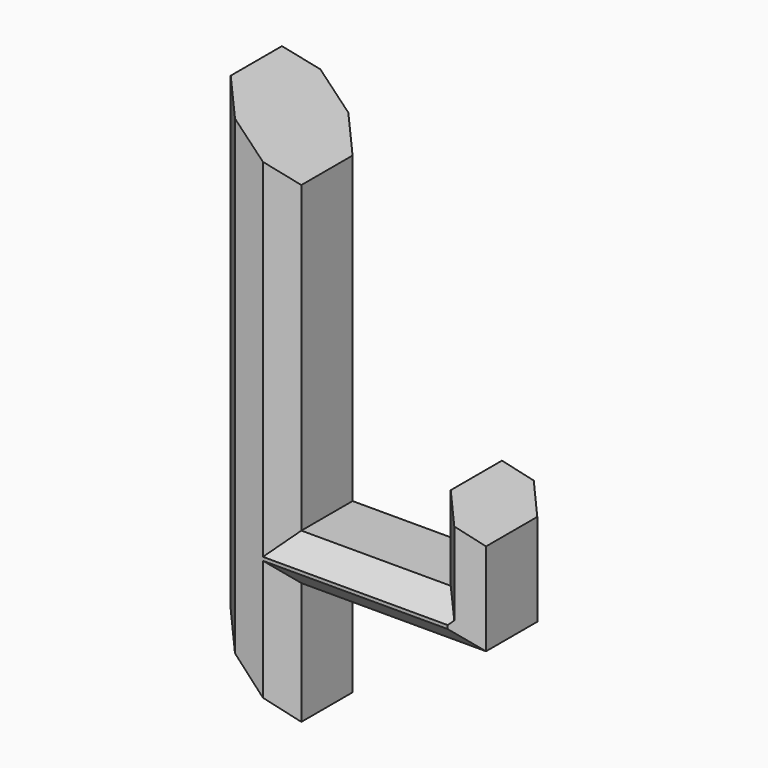
from build123d import *

# Parameters (mm, degrees)
F1_DEPTH   = 25
F2_SIZE    = 5
F3_SIZE    = 5
F4_C1_SIZE = 5
F4_C2_SIZE = 5
F4_C3_SIZE = 5
F4_C4_SIZE = 5
F5_SIZE    = 5
F6_R       = 3.8134977221
F6_R_2     = 4.2636207358
F6_R_3     = 3.889016134
F6_R_4     = 3.7558552916
F6_R_5     = 4.5761931688
F6_R_6     = 1.7054444875
F7_DEPTH   = 2.5


with BuildPart() as f1:
    # F0 (on Front) → F1 (new body)
    with BuildSketch(Plane.XZ):
        Polygon((0, 0), (0, 21.6363706006), (-8.27272566, 30.5454584579), (-8.27272566, 10.8181868544), (-43.27272566, 10.8181868544), (-43.27272566, 0), align=None)
        Polygon((-43.27272566, -28.6363649917), (-43.27272566, 0), (-43.27272566, 10.8181868544), (-43.27272566, 82.0909227153), (-59.8181864452, 99.2727460619), (-59.8181864452, -10.8181790838), align=None)
    extrude(amount=F1_DEPTH)

    # F2
    f2_edges = [f1.edges().sort_by_distance(p)[0] for p in [
        (-25.772726, -25, 10.818187),
        (-21.636363, -25, 0),
    ]]
    chamfer(f2_edges, length=F2_SIZE)

    # F3
    f3_edges = [f1.edges().sort_by_distance(p)[0] for p in [
        (-25.772726, 0, 10.818187),
        (-21.636363, 0, 0),
    ]]
    chamfer(f3_edges, length=F3_SIZE)

    # F4: chamfer of 5 on 4 edges, made by hand

    # F4_c1
    f4_c1_edges = [f1.edges().sort_by_distance(p)[0] for p in [
        (-8.27272566, 0, 20.6818226561),
        (-8.27272566, 0, 8.3181868544),
    ]]
    chamfer(f4_c1_edges, length=F4_C1_SIZE)

    # F4_c2
    f4_c2_edges = [f1.edges().sort_by_distance(p)[0] for p in [
        (-8.27272566, -25, 20.6818226561),
        (-8.27272566, -25, 8.3181868544),
    ]]
    chamfer(f4_c2_edges, length=F4_C2_SIZE)

    # F4_c3
    f4_c3_edges = [f1.edges().sort_by_distance(p)[0] for p in [
        (0, 0, 13.3181853003),
    ]]
    chamfer(f4_c3_edges, length=F4_C3_SIZE)

    # F4_c4
    f4_c4_edges = [f1.edges().sort_by_distance(p)[0] for p in [
        (0, -25, 13.3181853003),
    ]]
    chamfer(f4_c4_edges, length=F4_C4_SIZE)

    # F5
    f5_edges = [f1.edges().sort_by_distance(p)[0] for p in [
        (-43.272726, 0, 46.454555),
        (-43.272726, 0, -14.318182),
        (-59.818186, 0, 44.227283),
        (-43.272726, -25, 46.454555),
        (-43.272726, -25, -14.318182),
        (-59.818186, -25, 44.227283),
    ]]
    chamfer(f5_edges, length=F5_SIZE)

    # F6 (on face) → F7 (cut)
    with BuildSketch(Plane(origin=(-59.8181864452, 0, 0), x_dir=(0, -1, 0), z_dir=(-1, 0, 0))):
        with Locations((12.1186533943, 85.4130089283)):
            Circle(F6_R)
        with Locations((12.1186533943, 65.2014911175)):
            Circle(F6_R_2)
        with Locations((12.1186533943, 45.3713275492)):
            Circle(F6_R_3)
        with Locations((12.1186533943, 23.6344132572)):
            Circle(F6_R_4)
        with Locations((12.1186533943, 6.4736939967)):
            Circle(F6_R_5)
        with Locations((12.1186533943, -4.9667861313)):
            Circle(F6_R_6)
    extrude(amount=-F7_DEPTH, mode=Mode.SUBTRACT)


solid = f1.part
